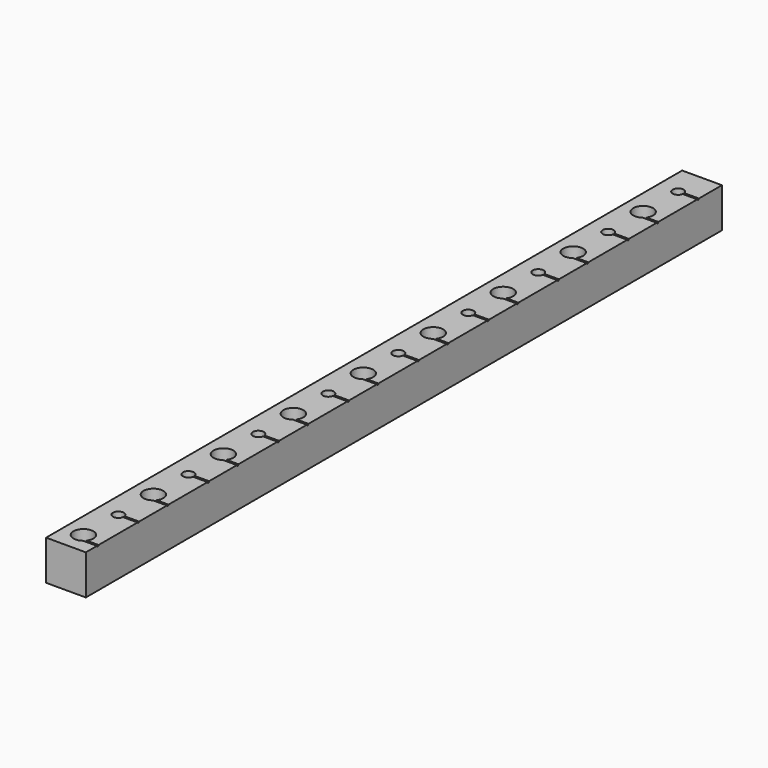
from build123d import *

# Parameters (mm, degrees)
F0_W     = 400
F0_H     = 20
F1_DEPTH = 20
F3_D     = 5.5
F3_DEPTH = 20
F3_TIP   = 1.6523667023
F5_D     = 10
F5_DEPTH = 20
F5_TIP   = 3.0043030951
F7_DEPTH = 10


# Not quite as in the source:
# - a feature names something its author has since deleted; it is built from what else it names


with BuildPart() as f1:
    # F0 (on Right) → F1 (new body)
    with BuildSketch(Plane.YZ):
        Rectangle(F0_W, F0_H)
    extrude(amount=F1_DEPTH)

    # F3
    with Locations(Plane.XY.offset(10)):
        with Locations((10, 185), (10, 141), (10, 97), (10, -167), (10, -123), (10, -79), (10, -35), (10, 9), (10, 53)):
            Hole(F3_D / 2, depth=F3_DEPTH)
            with Locations((0, 0, -(F3_DEPTH + F3_TIP / 2))):  # 118° drill point
                Cone(0, F3_D / 2, F3_TIP, mode=Mode.SUBTRACT)

    # F5
    with Locations(Plane.XY.offset(10)):
        with Locations((10, 163), (10, 119), (10, 75), (10, -189), (10, -145), (10, -101), (10, -57), (10, -13), (10, 31)):
            Hole(F5_D / 2, depth=F5_DEPTH)
            with Locations((0, 0, -(F5_DEPTH + F5_TIP / 2))):  # 118° drill point
                Cone(0, F5_D / 2, F5_TIP, mode=Mode.SUBTRACT)

    # F6 (on face) → F7 (cut)
    with BuildSketch(Plane.YZ.offset(20)):
        with BuildLine():
            ThreePointArc((71, 10), (71.5, 9.5), (72, 10))
            Line((72, 10), (71, 10))
        make_face()
        with BuildLine():
            ThreePointArc((96.5, 10), (97, 9.5), (97.5, 10))
            Line((97.5, 10), (96.5, 10))
        make_face()
        with BuildLine():
            ThreePointArc((115, 10), (115.5, 9.5), (116, 10))
            Line((116, 10), (115, 10))
        make_face()
        with BuildLine():
            ThreePointArc((140.5, 10), (141, 9.5), (141.5, 10))
            Line((141.5, 10), (140.5, 10))
        make_face()
        with BuildLine():
            ThreePointArc((159, 10), (159.5, 9.5), (160, 10))
            Line((160, 10), (159, 10))
        make_face()
        with BuildLine():
            Line((185.5, 10), (184.5, 10))
            ThreePointArc((184.5, 10), (185, 9.5), (185.5, 10))
        make_face()
        with BuildLine():
            ThreePointArc((52.5, 10), (53, 9.5), (53.5, 10))
            Line((53.5, 10), (52.5, 10))
        make_face()
        with BuildLine():
            ThreePointArc((27, 10), (27.5, 9.5), (28, 10))
            Line((28, 10), (27, 10))
        make_face()
        with BuildLine():
            ThreePointArc((8.5, 10), (9, 9.5), (9.5, 10))
            Line((9.5, 10), (8.5, 10))
        make_face()
        with BuildLine():
            ThreePointArc((-17, 10), (-16.5, 9.5), (-16, 10))
            Line((-16, 10), (-17, 10))
        make_face()
        with BuildLine():
            ThreePointArc((-35.5, 10), (-35, 9.5), (-34.5, 10))
            Line((-34.5, 10), (-35.5, 10))
        make_face()
        with BuildLine():
            Line((-60, 10), (-61, 10))
            ThreePointArc((-61, 10), (-60.5, 9.5), (-60, 10))
        make_face()
        with BuildLine():
            Line((-78.5, 10), (-79.5, 10))
            ThreePointArc((-79.5, 10), (-79, 9.5), (-78.5, 10))
        make_face()
        with BuildLine():
            Line((-104, 10), (-105, 10))
            ThreePointArc((-105, 10), (-104.5, 9.5), (-104, 10))
        make_face()
        with BuildLine():
            Line((-122.5, 10), (-123.5, 10))
            ThreePointArc((-123.5, 10), (-123, 9.5), (-122.5, 10))
        make_face()
        with BuildLine():
            Line((-148, 10), (-149, 10))
            ThreePointArc((-149, 10), (-148.5, 9.5), (-148, 10))
        make_face()
        with BuildLine():
            Line((-166.5, 10), (-167.5, 10))
            ThreePointArc((-167.5, 10), (-167, 9.5), (-166.5, 10))
        make_face()
        with BuildLine():
            Line((-192, 10), (-193, 10))
            ThreePointArc((-193, 10), (-192.5, 9.5), (-192, 10))
        make_face()
    extrude(amount=-F7_DEPTH, mode=Mode.SUBTRACT)


solid = f1.part
